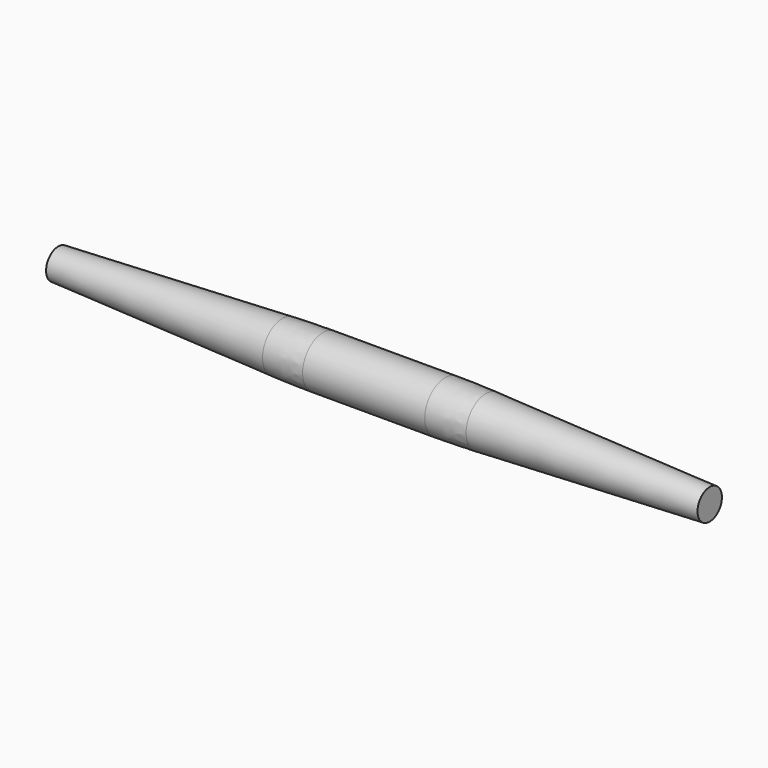
from build123d import *


# Not quite as in the source:
# - a fillet or chamfer that OpenCascade refuses, or shapes differently, is made with other operations: its cross-section is extruded or revolved along the edge and cut away or added


with BuildPart() as f1:
    # F0 (on Front) → F1 (revolve)
    with BuildSketch(Plane.XZ):
        Polygon((0, 9.525), (0, 0), (406.4, 0), (406.4, 9.525), (254, 15.875), (152.4, 15.875), align=None)
    revolve(axis=Axis((203.2, 0, 0), (1, 0, 0)))

    # F2: fillet of radius 609.6 on 2 edges, made by hand

    # F2_s1 → F2_t2 (revolve, cut)
    with BuildSketch(Plane.XZ):
        with BuildLine():
            ThreePointArc((165.0944926269, 15.875), (152.4027515975, 15.7428660189), (139.7165125703, 15.3465213571))
            Line((139.7165125703, 15.3465213571), (152.4, 15.875))
            Line((152.4, 15.875), (165.0944926269, 15.875))
        make_face()
    revolve(axis=Axis((152.4, 0, 0), (1, 0, 0)), mode=Mode.SUBTRACT)

    # F2_s3 → F2_t4 (revolve, cut)
    with BuildSketch(Plane.XZ):
        with BuildLine():
            ThreePointArc((266.6834874297, 15.3465213571), (253.9972484025, 15.7428660189), (241.3055073731, 15.875))
            Line((241.3055073731, 15.875), (254, 15.875))
            Line((254, 15.875), (266.6834874297, 15.3465213571))
        make_face()
    revolve(axis=Axis((254, 0, 0), (1, 0, 0)), mode=Mode.SUBTRACT)


solid = f1.part
